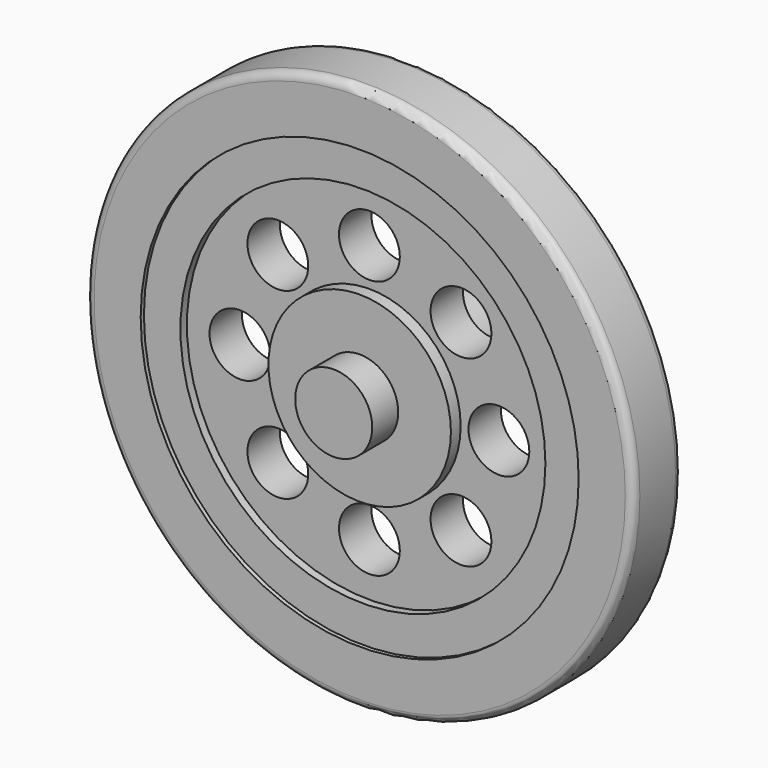
from build123d import *

# Parameters (mm, degrees)
F0_R      = 17.145
F1_DEPTH  = 3.81
F2_R      = 13.716
F2_R_2    = 11.43
F3_DEPTH  = 0.254
F4_DEPTH  = 0.762
F5_R      = 5.715
F6_DEPTH  = 0.762
F8_R      = 1.905
F9_DEPTH  = 25.4
F10_R     = 2.413
F11_DEPTH = 2.032
F14_R     = 3.175
F15_DEPTH = 8.89
F16_R     = 1.905
F17_DEPTH = 8.89
F18_R     = 0.508
F19_R     = 0.508
F20_R     = 13.208
F20_R_2   = 10.668
F21_DEPTH = 0.254
F22_DEPTH = 0.508


# Not quite as in the source:
# - the program builds the solid bodies; features that only make, move or delete a surface that nothing else refers to are left out


with BuildPart() as f1:
    # F0 (on Front) → F1 (new body)
    with BuildSketch(Plane.XZ):
        Circle(F0_R)
    extrude(amount=F1_DEPTH)

    # F2 (on face) → F3 (cut)
    with BuildSketch(Plane.XZ.offset(3.81)):
        Circle(F2_R)
        Circle(F2_R_2, mode=Mode.SUBTRACT)
    extrude(amount=-F3_DEPTH, mode=Mode.SUBTRACT)

    # F4 (cut): a face of the model
    f4_faces = [f1.faces().sort_by_distance(p)[0] for p in [
        (0, -3.81, 0),
    ]]
    extrude(f4_faces, amount=-F4_DEPTH, mode=Mode.SUBTRACT)

    # F5 (on face) → F6 (join)
    with BuildSketch(Plane.XZ.offset(3.048)):
        Circle(F5_R)
    extrude(amount=F6_DEPTH)

    # F8 (on face) → F9 (cut)
    with BuildSketch(Plane.XZ.offset(3.048)):
        with Locations((0, 8.1100180022)):
            Circle(F8_R)
        with Locations((-5.7346487249, 5.7346487249)):
            Circle(F8_R)
        with Locations((-5.7346487249, -5.7346487249)):
            Circle(F8_R)
        with Locations((0, -8.1100180022)):
            Circle(F8_R)
        with Locations((5.7346487249, -5.7346487249)):
            Circle(F8_R)
        with Locations((8.1100180022, 0)):
            Circle(F8_R)
        with Locations((5.7346487249, 5.7346487249)):
            Circle(F8_R)
        with Locations((-8.1100180022, 0)):
            Circle(F8_R)
    extrude(amount=-F9_DEPTH, mode=Mode.SUBTRACT)

    # F10 (on face) → F11 (join)
    with BuildSketch(Plane.XZ.offset(3.81)):
        Circle(F10_R)
    extrude(amount=F11_DEPTH)

    # F14 (on Front) → F15 (join)
    with BuildSketch(Plane.XZ):
        Circle(F14_R)
    extrude(amount=-F15_DEPTH)

    # F16 (on face) → F17 (cut)
    with BuildSketch(Plane(origin=(0, 8.89, 0), x_dir=(-1, 0, 0), z_dir=(0, 1, 0))):
        Circle(F16_R)
    extrude(amount=-F17_DEPTH, mode=Mode.SUBTRACT)

    # F18
    f18_edges = [f1.edges().sort_by_distance(p)[0] for p in [
        (-17.145, -3.81, 0),
    ]]
    fillet(f18_edges, radius=F18_R)

    # F19
    f19_edges = [f1.edges().sort_by_distance(p)[0] for p in [
        (-17.145, 0, 0),
    ]]
    fillet(f19_edges, radius=F19_R)

    # F20 (on face) → F21 (cut)
    with BuildSketch(Plane(origin=(0, 0, 0), x_dir=(-1, 0, 0), z_dir=(0, 1, 0))):
        Circle(F20_R)
        Circle(F20_R_2, mode=Mode.SUBTRACT)
    extrude(amount=-F21_DEPTH, mode=Mode.SUBTRACT)

    # F22 (cut): a face of the model
    f22_faces = [f1.faces().sort_by_distance(p)[0] for p in [
        (10.3662633943, 0, 0),
    ]]
    extrude(f22_faces, amount=-F22_DEPTH, mode=Mode.SUBTRACT)


solid = f1.part
